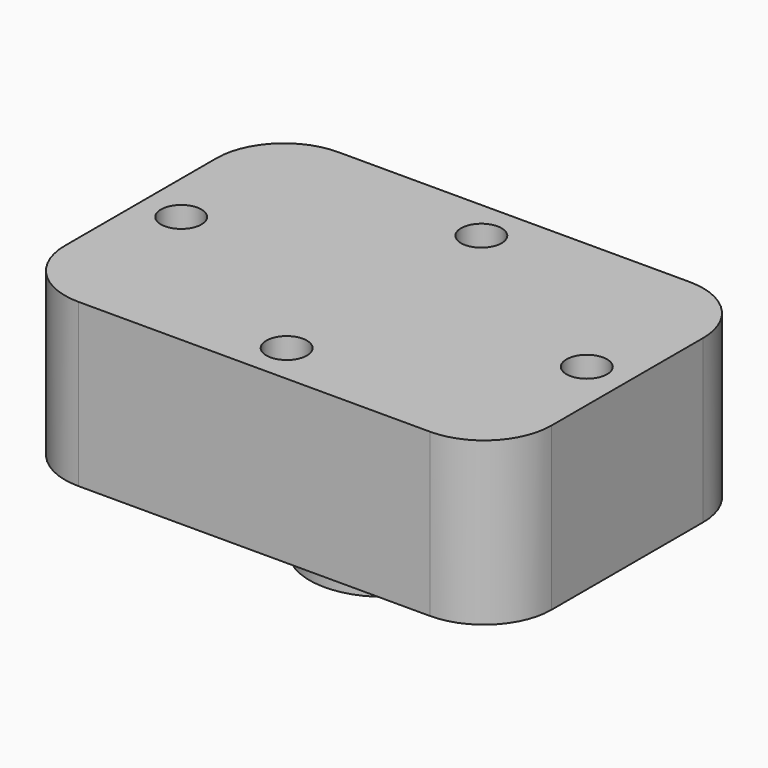
from build123d import *

# Parameters (mm, degrees)
F0_R     = 5.5
F0_R_2   = 4
F1_DEPTH = 12
F2_D     = 3
F3_R     = 2.5
F3_R_2   = 1.5
F4_DEPTH = 12
F6_DEPTH = 5


# Not quite as in the source:
# - a feature of the source that left no trace in its solid (it failed there, or was rolled back) is left out


with BuildPart() as f1:
    # F0 (on Top) → F1 (new body)
    with BuildSketch(Plane.XY):
        with BuildLine():
            Line((13, 12), (-13, 12))
            ThreePointArc((-13, 12), (-16.5355339059, 10.5355339059), (-18, 7))
            Line((-18, 7), (-18, -7))
            ThreePointArc((-18, -7), (-16.5355339059, -10.5355339059), (-13, -12))
            Line((-13, -12), (13, -12))
            ThreePointArc((13, -12), (16.5355339059, -10.5355339059), (18, -7))
            Line((18, -7), (18, 7))
            ThreePointArc((18, 7), (16.5355339059, 10.5355339059), (13, 12))
        make_face()
        Circle(F0_R, mode=Mode.SUBTRACT)
        Circle(F0_R)
        Circle(F0_R_2, mode=Mode.SUBTRACT)
        Circle(F0_R_2)
    extrude(amount=F1_DEPTH)

    # F2 (through all)
    with Locations(Plane(origin=(0, 0, 0), x_dir=(1, 0, 0), z_dir=(0, 0, -1))):
        with Locations((15, 0), (0, 9), (0, -9), (-15, 0)):
            Hole(F2_D / 2)

    # F3 (on face) → F4 (join, through all)
    with BuildSketch(Plane.XY):
        with Locations((0, 9)):
            Circle(F3_R)
        with Locations((0, 9)):
            Circle(F3_R_2, mode=Mode.SUBTRACT)
        with Locations((0, -9)):
            Circle(F3_R)
        with Locations((0, -9)):
            Circle(F3_R_2, mode=Mode.SUBTRACT)
    extrude(amount=F4_DEPTH)

    # F0 (on Top) → F6 (join)
    with BuildSketch(Plane.XY):
        Circle(F0_R)
        Circle(F0_R_2, mode=Mode.SUBTRACT)
    extrude(amount=-F6_DEPTH)


solid = f1.part
